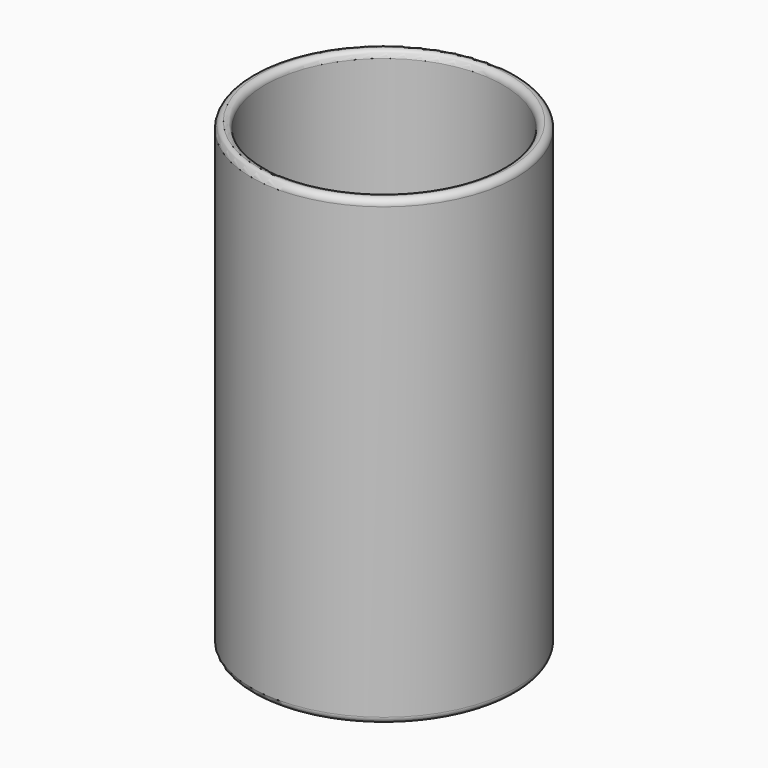
from build123d import *

# Parameters (mm, degrees)
F0_W = 2
F0_H = 70
F2_R = 0.99999


# Not quite as in the source:
# - a fillet or chamfer is up to 0.001 mm smaller than in the source, because OpenCascade refuses the exact size


with BuildPart() as f1:
    # F0 (on Front) → F1 (revolve)
    with BuildSketch(Plane.XZ):
        with Locations((-7.899047263, 13.5642557819)):
            Rectangle(F0_W, F0_H)
    revolve(axis=Axis((11.100952737, 0, 13.5642557819), (0, 0, -1)))

    # F2 (radius 1 in the source; OpenCascade refuses exactly that, so slightly less here)
    f2_edges = [f1.edges().sort_by_distance(p)[0] for p in [
        (29.100953, 0, 48.564256),
        (31.100953, 0, 48.564256),
        (31.100953, 0, -21.435744),
        (29.100953, 0, -21.435744),
    ]]
    fillet(f2_edges, radius=F2_R)


solid = f1.part
